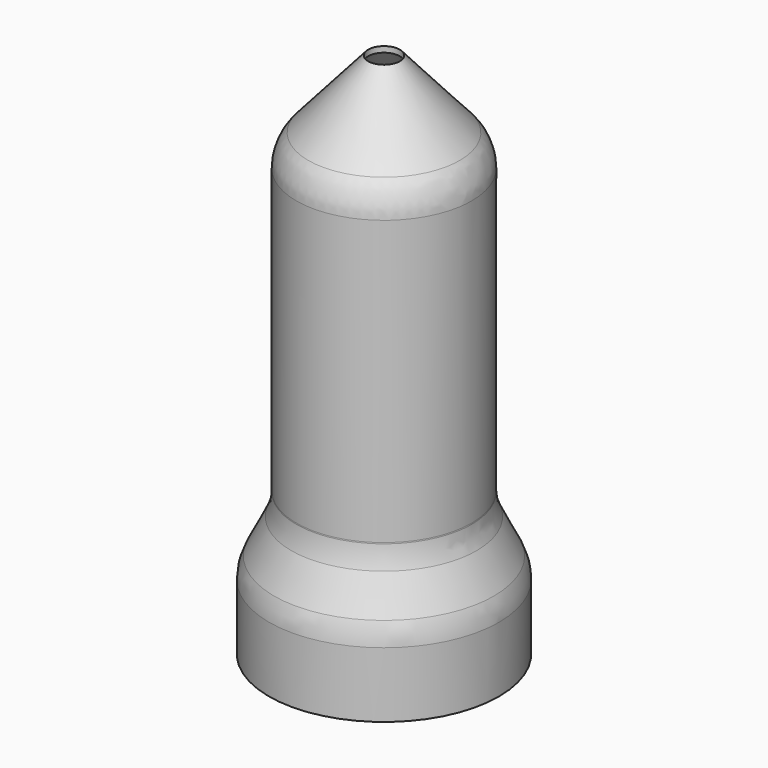
from build123d import *

# Parameters (mm, degrees)
F0_R        = 18.3
F1_DEPTH    = 110
F0_R_2      = 24
F0_R_3      = 19.5
F2_DEPTH    = 30
F3_S5_R     = 18.3
F3_T6_DEPTH = 36
F4_SIZE2    = 17
F4_SIZE     = 15
F5_R        = 10
F6_T        = -0.8
F7_DEPTH    = 25


# Not quite as in the source:
# - a fillet or chamfer that OpenCascade refuses, or shapes differently, is made with other operations: its cross-section is extruded or revolved along the edge and cut away or added


with BuildPart() as f1:
    # F0 (on Top) → F1 (new body)
    with BuildSketch(Plane.XY):
        Circle(F0_R)
    extrude(amount=F1_DEPTH)

    # F0 (on Top) → F2 (join)
    with BuildSketch(Plane.XY):
        Circle(F0_R_2)
        Circle(F0_R_3, mode=Mode.SUBTRACT)
        Circle(F0_R_3)
        Circle(F0_R, mode=Mode.SUBTRACT)
    extrude(amount=F2_DEPTH)

    # F3: chamfer of 7 x 14 on 1 edges, made by hand


with BuildPart() as f3_tool2:
    # F3_s3 → F3_t4 (revolve)
    with BuildSketch(Plane.XZ):
        Polygon((17, 30), (24, 16), (24, 30), align=None)
    revolve(axis=Axis((0, 0, 30), (0, 0, 1)))

    # F3_s5 → F3_t6 (cut, symmetric)
    with BuildSketch(Plane.XY.offset(23)):
        Circle(F3_S5_R)
    extrude(amount=F3_T6_DEPTH, both=True, mode=Mode.SUBTRACT)


with BuildPart() as f1_1:
    add(f1.part)

    # F3_t1: cut F3_tool2
    add(f3_tool2.part, mode=Mode.SUBTRACT)

    # F4
    f4_edges = [f1_1.edges().sort_by_distance(p)[0] for p in [
        (-18.3, 0, 110),
    ]]
    f4_side = f1_1.faces().sort_by_distance((0, 0, 110))[0]
    chamfer(f4_edges, length=F4_SIZE, length2=F4_SIZE2, reference=f4_side)

    # F5
    f5_edges = [f1_1.edges().sort_by_distance(p)[0] for p in [
        (-18.3, 0, 93),
        (-18.3, 0, 30),
        (-18.3, 0, 27.4),
        (-24, 0, 16),
    ]]
    fillet(f5_edges, radius=F5_R)

    # F6
    f6_openings = [f1_1.faces().sort_by_distance(p)[0] for p in [
        (0, 0, 0),
    ]]
    offset(amount=F6_T, openings=f6_openings)

    # F7 (cut): a face of the model
    f7_faces = [f1_1.faces().sort_by_distance(p)[0] for p in [
        (0, 0, 110),
    ]]
    extrude(f7_faces, amount=-F7_DEPTH, mode=Mode.SUBTRACT)


solid = f1_1.part
